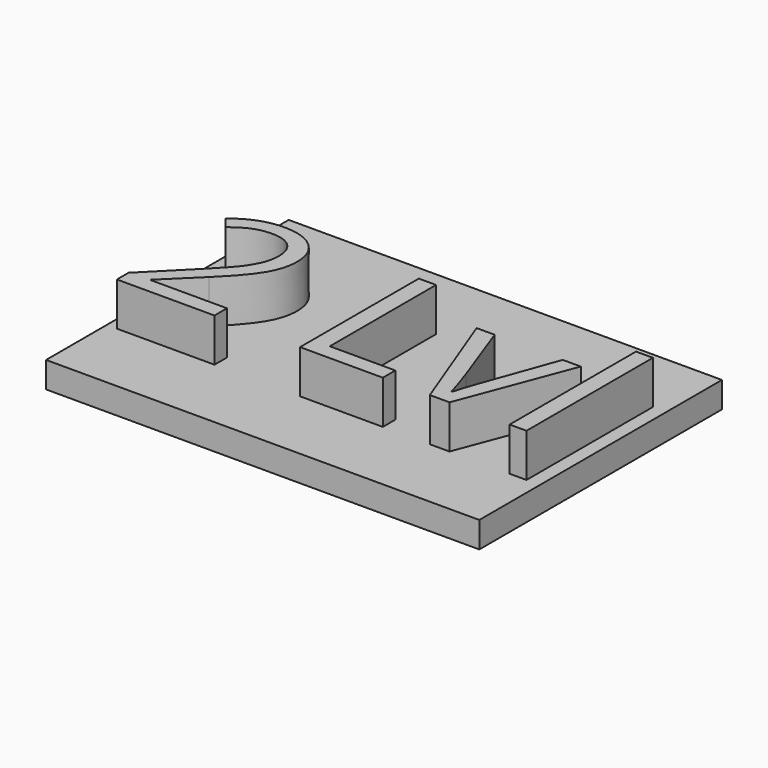
from build123d import *

# Parameters (mm, degrees)
F0_W         = 20
F0_H         = 14
F1_DEPTH     = 1.2
F2_TEXT_SIZE = 9.599520024
F3_DEPTH     = 2


# Not quite as in the source:
# - Text() gives the source's letters only with a copy of the font that has no kerning and outlines rounded to 1/6400 em; it was checked with that copy


with BuildPart() as f1:
    # F0 (on Top) → F1 (new body)
    with BuildSketch(Plane.XY):
        with Locations((10, 7)):
            Rectangle(F0_W, F0_H)
    extrude(amount=F1_DEPTH)

    # F2 (on face) → F3 (join)
    with BuildSketch(Plane.XY.offset(1.2)):
        with Locations((0, 3.5)):
            Text('2 Lvl', F2_TEXT_SIZE, font='Open Sans', text_align=(TextAlign.LEFT, TextAlign.BOTTOM))
    extrude(amount=F3_DEPTH)


solid = f1.part
